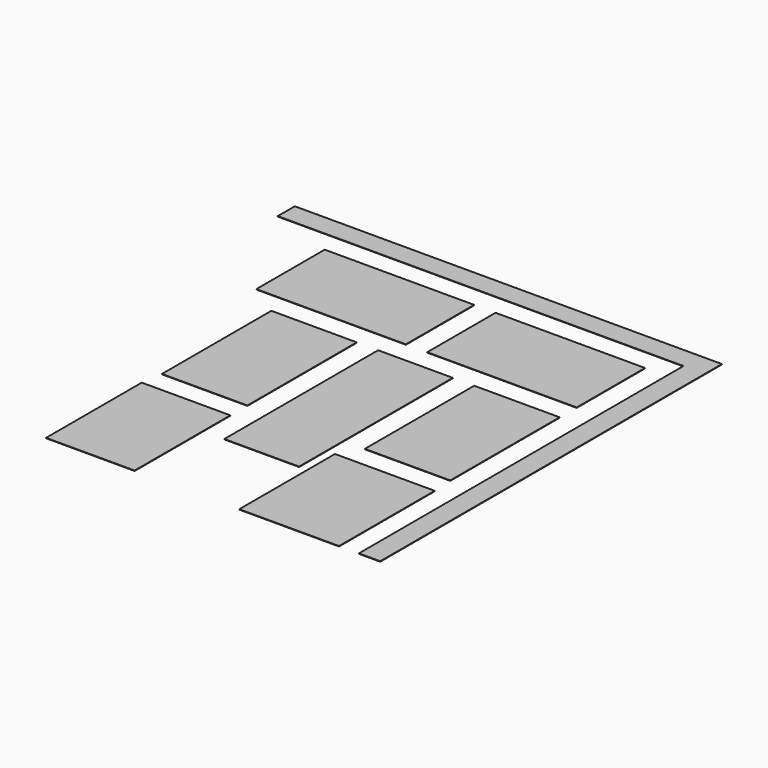
from build123d import *

# Parameters (mm, degrees)
F2_W     = 2073.7516880035
F2_H     = 2800
F3_DEPTH = 10
F2_W_2   = 2335.388469696
F2_W_3   = 1750
F2_H_2   = 4500
F2_W_4   = 2000
F2_H_3   = 3200
F2_W_5   = 3500
F2_H_4   = 2000
F4_DEPTH = 10


# Not quite as in the source:
# - the program builds the solid bodies; features that only make, move or delete a surface that nothing else refers to are left out


with BuildPart() as f3:
    # F2 (on face) → F3 (new body)
    with BuildSketch(Plane.XY):
        with Locations((-1786.8758440018, -3600)):
            Rectangle(F2_W, F2_H)
    extrude(amount=F3_DEPTH)


with BuildPart() as f3b:
    # F2 (on face) → F3, piece 2 (new body)
    with BuildSketch(Plane.XY):
        with Locations((2867.694234848, -3600)):
            Rectangle(F2_W_2, F2_H)
    extrude(amount=F3_DEPTH)


with BuildPart() as f3c:
    # F2 (on face) → F3, piece 3 (new body)
    with BuildSketch(Plane.XY):
        with Locations((625, -750)):
            Rectangle(F2_W_3, F2_H_2)
    extrude(amount=F3_DEPTH)


with BuildPart() as f3d:
    # F2 (on face) → F3, piece 4 (new body)
    with BuildSketch(Plane.XY):
        with Locations((3000, -100)):
            Rectangle(F2_W_4, F2_H_3)
    extrude(amount=F3_DEPTH)


with BuildPart() as f3e:
    # F2 (on face) → F3, piece 5 (new body)
    with BuildSketch(Plane.XY):
        with Locations((-1750, -100)):
            Rectangle(F2_W_4, F2_H_3)
    extrude(amount=F3_DEPTH)


with BuildPart() as f3f:
    # F2 (on face) → F3, piece 6 (new body)
    with BuildSketch(Plane.XY):
        with Locations((-1750, 3000)):
            Rectangle(F2_W_5, F2_H_4)
    extrude(amount=F3_DEPTH)


with BuildPart() as f3g:
    # F2 (on face) → F3, piece 7 (new body)
    with BuildSketch(Plane.XY):
        with Locations((2250, 3000)):
            Rectangle(F2_W_5, F2_H_4)
    extrude(amount=F3_DEPTH)


with BuildPart() as f4:
    # F1 (on face) → F4 (new body)
    with BuildSketch(Plane.XY):
        Polygon((4500, 4500), (4500, -5000), (5000, -5000), (5000, 5000), (-5000, 5000), (-5000, 4500), align=None)
    extrude(amount=F4_DEPTH)


solid = Compound([f3.part, f3b.part, f3c.part, f3d.part, f3e.part, f3f.part, f3g.part, f4.part])
